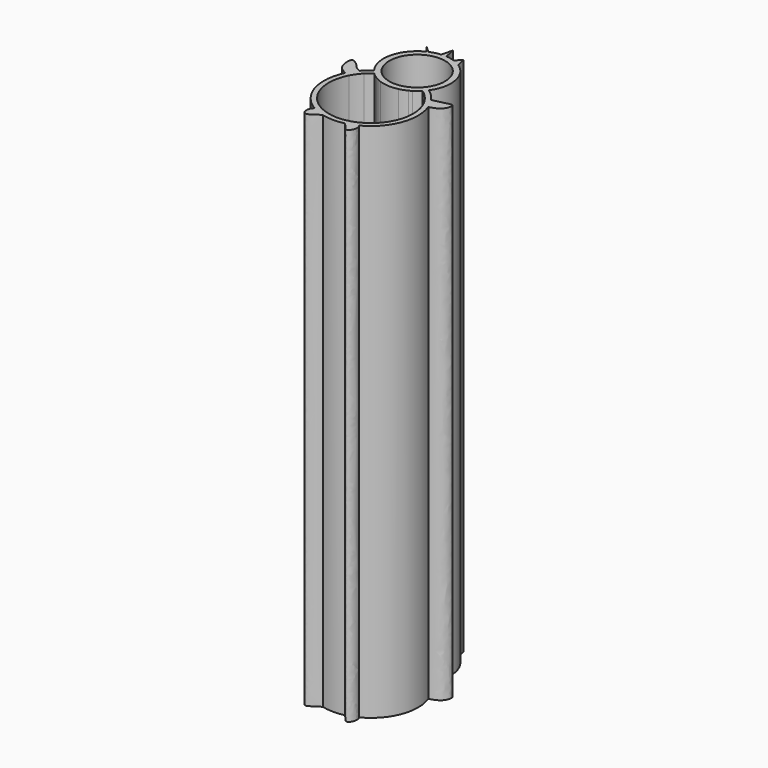
from build123d import *

# Parameters (mm, degrees)
F0_R     = 1.3574899336
F1_DEPTH = 25.4


with BuildPart() as f1:
    # F0 (on Top) → F1 (new body)
    with BuildSketch(Plane.XY):
        with BuildLine():
            Line((35.2878831327, 25.0843970505), (35.0384411812, 24.8051633126))
            ThreePointArc((35.0384411812, 24.8051633126), (34.8900331306, 24.8498952124), (34.7380711454, 24.8804475838))
            ThreePointArc((34.7380711454, 24.8804475838), (34.6718324932, 24.8891687339), (34.6052941294, 24.8951906649))
            ThreePointArc((34.6052941294, 24.8951906649), (34.4790949379, 24.8991686132), (34.3529627664, 24.8934471338))
            ThreePointArc((34.3529627664, 24.8934471338), (34.0864715287, 24.84878651), (33.8308991876, 24.7610657624))
            ThreePointArc((33.8308991876, 24.7610657624), (33.7935953989, 24.7441653158), (33.7567242747, 24.7263406713))
            ThreePointArc((33.7567242747, 24.7263406713), (32.8919741005, 23.6379870392), (33.1706458564, 22.2761322214))
            ThreePointArc((33.1706458564, 22.2761322214), (33.2477936638, 22.1799429615), (33.331935669, 22.0898081689))
            ThreePointArc((33.331935669, 22.0898081689), (33.4714507341, 21.9660817612), (33.624082862, 21.8589551498))
            ThreePointArc((33.624082862, 21.8589551498), (33.6972022109, 21.8161682858), (33.7724291489, 21.7772059613))
            ThreePointArc((33.7724291489, 21.7772059613), (33.8523875779, 21.7409790551), (33.9341661368, 21.7090728424))
            add(Edge.make_bspline(
                [(34.8690945447, 21.6562799961), (34.5503462489, 21.6638848484), (34.2300963573, 21.682290249), (33.9341661368, 21.7090728424)],
                knots=[0.8742249562, 0.8742249562, 0.8742249562, 0.8742249562, 0.9209885647, 0.9209885647, 0.9209885647, 0.9209885647], degree=3))
            ThreePointArc((34.8690945447, 21.6562799961), (35.054677069, 21.7119521289), (35.2324185413, 21.7890768896))
            ThreePointArc((35.2324185413, 21.7890768896), (35.3070019831, 21.8292572971), (35.3794159251, 21.8732274679))
            ThreePointArc((35.3794159251, 21.8732274679), (35.5302859315, 21.982821804), (35.6677706867, 22.1088004507))
            ThreePointArc((35.6677706867, 22.1088004507), (35.7504359225, 22.200291525), (35.826009436, 22.2977225363))
            ThreePointArc((35.826009436, 22.2977225363), (36.1066779775, 23.5541858288), (35.3956624922, 24.6274666939))
            Line((35.3956624922, 24.6274666939), (35.2878831327, 25.0843970505))
        make_face()
        with Locations((34.4904512167, 23.2556387782)):
            Circle(F0_R, mode=Mode.SUBTRACT)
        Polygon((34.4900014006, 25.4237678916), (34.6052941294, 24.8951906649), (34.4904512167, 25.4255086183), align=None)
        with BuildLine():
            ThreePointArc((34.3529627664, 24.8934471338), (34.4790949379, 24.8991686132), (34.6052941294, 24.8951906649))
            Line((34.6052941294, 24.8951906649), (34.4900014006, 25.4237678916))
            Line((34.4900014006, 25.4237678916), (34.3529627664, 24.8934471338))
        make_face()
        with BuildLine():
            ThreePointArc((36.3961035597, 21.729501502), (36.1361243059, 22.0387624609), (35.826009436, 22.2977225363))
            ThreePointArc((35.826009436, 22.2977225363), (35.7504359225, 22.200291525), (35.6677706867, 22.1088004507))
            ThreePointArc((35.6677706867, 22.1088004507), (35.9078628578, 21.9178867809), (36.1168310715, 21.6933326324))
            add(Edge.make_bspline(
                [(36.3961035597, 21.729501502), (36.3090749695, 21.7153973416), (36.2155393433, 21.7033827965), (36.1168310715, 21.6933326324)],
                knots=[0.7920048431, 0.7920048431, 0.7920048431, 0.7920048431, 0.8094233051, 0.8094233051, 0.8094233051, 0.8094233051], degree=3))
        make_face()
        with BuildLine():
            ThreePointArc((33.7567242747, 24.7263406713), (33.7935953989, 24.7441653158), (33.8308991876, 24.7610657624))
            Line((33.8308991876, 24.7610657624), (33.4780786019, 25.0843970505))
            Line((33.4780786019, 25.0843970505), (33.7567242747, 24.7263406713))
        make_face()
        with BuildLine():
            add(Edge.make_bspline(
                [(36.6693598159, 21.2079252289), (37.0767596252, 21.3101548698), (37.3116579362, 21.5662061593), (37.3529850038, 22.0550492964), (36.9161573246, 21.8137832496), (36.3961035597, 21.729501502)],
                knots=[0.5386602181, 0.5386602181, 0.5386602181, 0.5386602181, 0.6339632831, 0.6879179364, 0.7920048431, 0.7920048431, 0.7920048431, 0.7920048431], degree=3))
            add(Edge.make_bspline(
                [(36.3961035597, 21.729501502), (36.3090749695, 21.7153973416), (36.2155393433, 21.7033827965), (36.1168310715, 21.6933326324)],
                knots=[0.7920048431, 0.7920048431, 0.7920048431, 0.7920048431, 0.8094233051, 0.8094233051, 0.8094233051, 0.8094233051], degree=3))
            ThreePointArc((36.1168310715, 21.6933326324), (36.2914503946, 21.437661713), (36.4256376999, 21.1586396813))
            add(Edge.make_bspline(
                [(36.4256376999, 21.1586396813), (36.5143437357, 21.1731050665), (36.5960224931, 21.1895225492), (36.6693598159, 21.2079252289)],
                knots=[0.5215044131, 0.5215044131, 0.5215044131, 0.5215044131, 0.5386602181, 0.5386602181, 0.5386602181, 0.5386602181], degree=3))
        make_face()
        with BuildLine():
            ThreePointArc((35.5719280309, 18.3706314653), (36.65722528, 19.581735003), (36.6693598159, 21.2079252289))
            add(Edge.make_bspline(
                [(36.4256376999, 21.1586396813), (36.5143437357, 21.1731050665), (36.5960224931, 21.1895225492), (36.6693598159, 21.2079252289)],
                knots=[0.5215044131, 0.5215044131, 0.5215044131, 0.5215044131, 0.5386602181, 0.5386602181, 0.5386602181, 0.5386602181], degree=3))
            ThreePointArc((36.4256376999, 21.1586396813), (36.4145776308, 19.6354161553), (35.3570595451, 18.5390641437))
            add(Edge.make_bspline(
                [(35.5719280309, 18.3706314653), (35.5261594748, 18.4364082043), (35.4517435721, 18.492565667), (35.3570595451, 18.5390641437)],
                knots=[0.7349975613, 0.7349975613, 0.7349975613, 0.7349975613, 0.7758927384, 0.7758927384, 0.7758927384, 0.7758927384], degree=3))
        make_face()
        with BuildLine():
            ThreePointArc((33.331935669, 22.0898081689), (33.2477936638, 22.1799429615), (33.1706458564, 22.2761322214))
            ThreePointArc((33.1706458564, 22.2761322214), (32.9577020916, 22.1025904709), (32.7669837029, 21.9048829033))
            add(Edge.make_bspline(
                [(33.0339498666, 21.8341794774), (32.9292845175, 21.856390058), (32.8391193359, 21.8800682788), (32.7669837029, 21.9048829033)],
                knots=[0.9759112078, 0.9759112078, 0.9759112078, 0.9759112078, 1, 1, 1, 1], degree=3))
            ThreePointArc((33.0339498666, 21.8341794774), (33.1768182667, 21.9691331407), (33.331935669, 22.0898081689))
        make_face()
        with BuildLine():
            add(Edge.make_bspline(
                [(35.0284066637, 18.1708643732), (35.2170583716, 18.0273126704), (35.3967964234, 17.5080415665), (35.724938715, 18.1507306273), (35.5719280309, 18.3706314653)],
                knots=[0.4666277679, 0.4666277679, 0.4666277679, 0.4666277679, 0.5982792648, 0.7349975613, 0.7349975613, 0.7349975613, 0.7349975613], degree=3))
            add(Edge.make_bspline(
                [(35.5719280309, 18.3706314653), (35.5261594748, 18.4364082043), (35.4517435721, 18.492565667), (35.3570595451, 18.5390641437)],
                knots=[0.7349975613, 0.7349975613, 0.7349975613, 0.7349975613, 0.7758927384, 0.7758927384, 0.7758927384, 0.7758927384], degree=3))
            ThreePointArc((35.3570595451, 18.5390641437), (34.4749160162, 18.3581603594), (33.6002109549, 18.5721567153))
            add(Edge.make_bspline(
                [(33.6002109549, 18.5721567153), (33.4997142497, 18.532511366), (33.4150808726, 18.4840593538), (33.3534064783, 18.426767052)],
                knots=[0.9613097376, 0.9613097376, 0.9613097376, 0.9613097376, 1, 1, 1, 1], degree=3))
            add(Edge.make_bspline(
                [(33.3534064783, 18.426767052), (33.1417874827, 18.2301840214), (33.2663690261, 17.591909312), (33.6656467439, 18.0441057117), (33.9492281969, 18.1828270385)],
                knots=[0, 0, 0, 0, 0.132755166, 0.2818249758, 0.2818249758, 0.2818249758, 0.2818249758], degree=3))
            add(Edge.make_bspline(
                [(33.9492281969, 18.1828270385), (34.3007859291, 18.3548007502), (34.7635911229, 18.3723718084), (35.0284066637, 18.1708643732)],
                knots=[0.2818249758, 0.2818249758, 0.2818249758, 0.2818249758, 0.4666277679, 0.4666277679, 0.4666277679, 0.4666277679], degree=3))
        make_face()
        with BuildLine():
            add(Edge.make_bspline(
                [(33.0339498666, 21.8341794774), (32.9292845175, 21.856390058), (32.8391193359, 21.8800682788), (32.7669837029, 21.9048829033)],
                knots=[0.9759112078, 0.9759112078, 0.9759112078, 0.9759112078, 1, 1, 1, 1], degree=3))
            add(Edge.make_bspline(
                [(32.7669837029, 21.9048829033), (32.5380625713, 21.9836316671), (32.4459364295, 22.1591315552), (31.9189267871, 22.595742553), (31.9114951341, 21.9415604187), (32.0737037979, 21.5876444724), (32.4533377986, 21.4297287765)],
                knots=[0, 0, 0, 0, 0.0764453478, 0.1487485697, 0.2171150564, 0.3144523622, 0.3144523622, 0.3144523622, 0.3144523622], degree=3))
            add(Edge.make_bspline(
                [(32.4533377986, 21.4297287765), (32.5223607921, 21.4010174018), (32.6007834055, 21.3739582167), (32.6871630664, 21.3485875551)],
                knots=[0.3144523622, 0.3144523622, 0.3144523622, 0.3144523622, 0.3321497028, 0.3321497028, 0.3321497028, 0.3321497028], degree=3))
            ThreePointArc((32.6871630664, 21.3485875551), (32.8428207036, 21.6040495599), (33.0339498666, 21.8341794774))
        make_face()
        with BuildLine():
            ThreePointArc((33.9341661368, 21.7090728424), (34.3977909817, 21.6146837622), (34.8690945447, 21.6562799961))
            add(Edge.make_bspline(
                [(34.8690945447, 21.6562799961), (34.5503462489, 21.6638848484), (34.2300963573, 21.682290249), (33.9341661368, 21.7090728424)],
                knots=[0.8742249562, 0.8742249562, 0.8742249562, 0.8742249562, 0.9209885647, 0.9209885647, 0.9209885647, 0.9209885647], degree=3))
        make_face()
        with BuildLine():
            ThreePointArc((33.9492281969, 18.1828270385), (34.4881053263, 18.1126052324), (35.0284066637, 18.1708643732))
            add(Edge.make_bspline(
                [(33.9492281969, 18.1828270385), (34.3007859291, 18.3548007502), (34.7635911229, 18.3723718084), (35.0284066637, 18.1708643732)],
                knots=[0.2818249758, 0.2818249758, 0.2818249758, 0.2818249758, 0.4666277679, 0.4666277679, 0.4666277679, 0.4666277679], degree=3))
        make_face()
        with BuildLine():
            add(Edge.make_bspline(
                [(32.4533377986, 21.4297287765), (32.5223607921, 21.4010174018), (32.6007834055, 21.3739582167), (32.6871630664, 21.3485875551)],
                knots=[0.3144523622, 0.3144523622, 0.3144523622, 0.3144523622, 0.3321497028, 0.3321497028, 0.3321497028, 0.3321497028], degree=3))
            ThreePointArc((32.4533377986, 21.4297287765), (32.3119414487, 19.7509801737), (33.3534064783, 18.426767052))
            add(Edge.make_bspline(
                [(33.6002109549, 18.5721567153), (33.4997142497, 18.532511366), (33.4150808726, 18.4840593538), (33.3534064783, 18.426767052)],
                knots=[0.9613097376, 0.9613097376, 0.9613097376, 0.9613097376, 1, 1, 1, 1], degree=3))
            ThreePointArc((33.6002109549, 18.5721567153), (32.5632602667, 19.7694949106), (32.6871630664, 21.3485875551))
        make_face()
    extrude(amount=F1_DEPTH)


solid = f1.part
